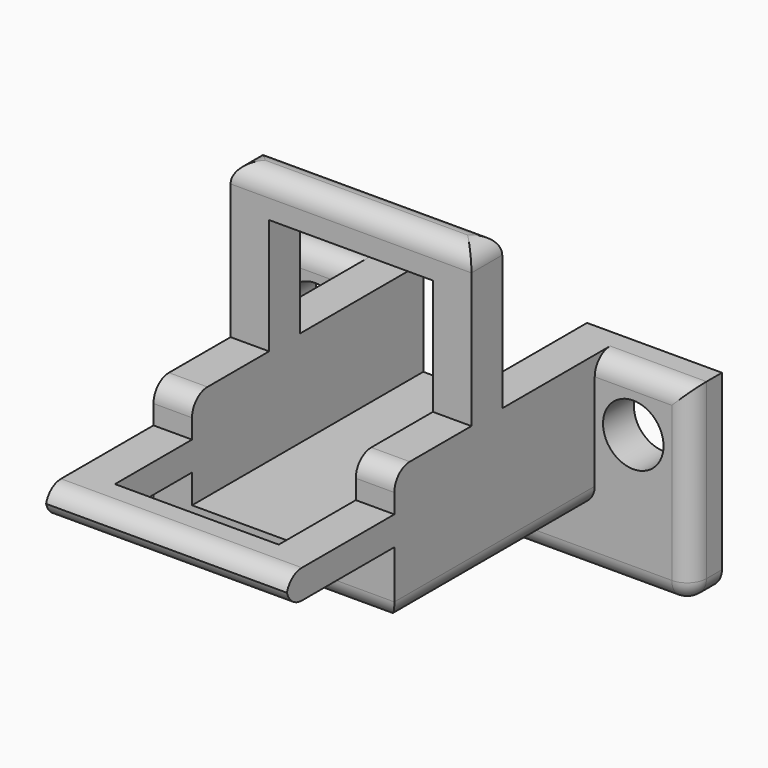
from build123d import *

# Parameters (mm, degrees)
F1_DEPTH      = 19.05
F0_R          = 1.9939
F2_DEPTH      = 2.54
F3_W          = 2.54
F3_H          = 1.905
F4_DEPTH      = 8.89
F5_W          = 2.54
F5_H          = 1.905
F6_DEPTH      = 11.43
F7_W          = 2.54
F7_H          = 2.54
F8_W          = 2.54
F8_H          = 2.54
F9_DEPTH      = 10.16
F10_W         = 2.54
F10_H         = 2.54
F11_DEPTH     = 11.43
F12_T1_DEPTH  = 9.525
F12_T3_DEPTH  = 14.605
F12_T5_DEPTH  = 26.035
F12_T7_DEPTH  = 9.525
F12_T9_DEPTH  = 4.445
F12_T11_DEPTH = 19.685
F12_T13_DEPTH = 22.225
F12_T15_DEPTH = 8.89
F12_T17_DEPTH = 8.89
F12_T19_DEPTH = 8.89
F12_S23_W     = 1.27
F12_S23_H     = 1.27
F12_T24_DEPTH = 1.27
F12_S29_W     = 1.27
F12_S29_H     = 1.27
F12_T30_DEPTH = 1.27


# Not quite as in the source:
# - a fillet or chamfer that OpenCascade refuses, or shapes differently, is made with other operations: its cross-section is extruded or revolved along the edge and cut away or added


with BuildPart() as f1:
    # F0 (on Front) → F1 (new body)
    with BuildSketch(Plane.XZ):
        Polygon((-23.2056408978, -6.35), (-23.2056408978, 0), (-25.7456408978, 0), (-25.7456408978, -8.89), (-9.8706408978, -8.89), (-9.8706408978, 0), (-12.4106408978, 0), (-12.4106408978, -6.35), align=None)
    extrude(amount=F1_DEPTH)

    # F0 (on Front) → F2 (join)
    with BuildSketch(Plane.XZ):
        Polygon((-25.7456408978, -8.89), (-25.7456408978, 0), (-32.0956408978, 0), (-32.0956408978, -12.7), (-3.5206408978, -12.7), (-3.5206408978, 0), (-9.8706408978, 0), (-9.8706408978, -8.89), align=None)
        Polygon((-28.6261399051, -11.2280230969), (-28.955778145, -11.2280230969), (-29.2968038878, -10.3571788012), (-30.3941995557, -10.3571788012), (-30.7310299027, -11.2280230969), (-31.0534760356, -11.2280230969), (-29.9710639241, -8.4782408335), (-29.7031579363, -8.4782408335), align=None, mode=Mode.SUBTRACT)
        with Locations((-28.2856408978, -3.81)):
            Circle(F0_R, mode=Mode.SUBTRACT)
        with Locations((-7.3306408978, -3.81)):
            Circle(F0_R, mode=Mode.SUBTRACT)
    extrude(amount=F2_DEPTH)

    # F3 (on face) → F4 (join)
    with BuildSketch(Plane.XZ.offset(19.05)):
        with Locations((-11.1406408978, -3.4925)):
            Rectangle(F3_W, F3_H)
        with Locations((-24.4756408978, -3.4925)):
            Rectangle(F3_W, F3_H)
    extrude(amount=F4_DEPTH)

    # F5 (on face) → F6 (join)
    with BuildSketch(Plane(origin=(-12.4106408978, 0, 0), x_dir=(0, -1, 0), z_dir=(-1, 0, 0))):
        with Locations((26.67, -3.4925)):
            Rectangle(F5_W, F5_H)
    extrude(amount=F6_DEPTH)

    # F7 (on face) + F8 (on face) → F9 (join)
    with BuildSketch(Plane.XY):
        with Locations((-24.4756408978, -11.43)):
            Rectangle(F7_W, F7_H)
    with BuildSketch(Plane.XY):
        with Locations((-11.1406408978, -11.43)):
            Rectangle(F8_W, F8_H)
    extrude(amount=F9_DEPTH)

    # F10 (on face) → F11 (join)
    with BuildSketch(Plane.YZ.offset(-23.2056408978)):
        with Locations((-11.43, 8.89)):
            Rectangle(F10_W, F10_H)
    extrude(amount=F11_DEPTH)

    # F12: fillet of radius 1.27 on 18 edges, made by hand

    # F12_s2 → F12_t1 (cut)
    with BuildSketch(Plane.YZ.offset(-35.2706408978)):
        with BuildLine():
            ThreePointArc((-1.27, 0), (-2.1680256121, -0.3719743879), (-2.54, -1.27))
            Line((-2.54, -1.27), (-2.54, 0))
            Line((-2.54, 0), (-1.27, 0))
        make_face()
    extrude(amount=F12_T1_DEPTH, mode=Mode.SUBTRACT)

    # F12_s4 → F12_t3 (cut)
    with BuildSketch(Plane.XY.offset(-11.43)):
        with BuildLine():
            ThreePointArc((-32.0956408978, -1.27), (-31.7236665099, -2.1680256121), (-30.8256408978, -2.54))
            Line((-30.8256408978, -2.54), (-32.0956408978, -2.54))
            Line((-32.0956408978, -2.54), (-32.0956408978, -1.27))
        make_face()
        with BuildLine():
            ThreePointArc((-3.5206408978, -1.27), (-3.8926152856, -2.1680256121), (-4.7906408978, -2.54))
            Line((-4.7906408978, -2.54), (-3.5206408978, -2.54))
            Line((-3.5206408978, -2.54), (-3.5206408978, -1.27))
        make_face()
    extrude(amount=F12_T3_DEPTH, mode=Mode.SUBTRACT)

    # F12_s6 → F12_t5 (cut)
    with BuildSketch(Plane.YZ.offset(-30.8256408978)):
        with BuildLine():
            ThreePointArc((-1.27, -12.7), (-2.1680256121, -12.3280256121), (-2.54, -11.43))
            Line((-2.54, -11.43), (-2.54, -12.7))
            Line((-2.54, -12.7), (-1.27, -12.7))
        make_face()
    extrude(amount=F12_T5_DEPTH, mode=Mode.SUBTRACT)

    # F12_s8 → F12_t7 (cut)
    with BuildSketch(Plane.YZ.offset(-9.8706408978)):
        with BuildLine():
            ThreePointArc((-1.27, 0), (-2.1680256121, -0.3719743879), (-2.54, -1.27))
            Line((-2.54, -1.27), (-2.54, 0))
            Line((-2.54, 0), (-1.27, 0))
        make_face()
    extrude(amount=F12_T7_DEPTH, mode=Mode.SUBTRACT)

    # F12_s10 → F12_t9 (cut)
    with BuildSketch(Plane.XZ.offset(-3.175)):
        with BuildLine():
            ThreePointArc((-4.7906408978, -12.7), (-3.8926152856, -12.3280256121), (-3.5206408978, -11.43))
            Line((-3.5206408978, -11.43), (-3.5206408978, -12.7))
            Line((-3.5206408978, -12.7), (-4.7906408978, -12.7))
        make_face()
        with BuildLine():
            ThreePointArc((-32.0956408978, -11.43), (-31.7236665099, -12.3280256121), (-30.8256408978, -12.7))
            Line((-30.8256408978, -12.7), (-32.0956408978, -12.7))
            Line((-32.0956408978, -12.7), (-32.0956408978, -11.43))
        make_face()
    extrude(amount=F12_T9_DEPTH, mode=Mode.SUBTRACT)

    # F12_s12 → F12_t11 (cut)
    with BuildSketch(Plane.XZ.offset(2.54)):
        with BuildLine():
            ThreePointArc((-9.8706408978, -7.62), (-10.2426152856, -8.5180256121), (-11.1406408978, -8.89))
            Line((-11.1406408978, -8.89), (-9.8706408978, -8.89))
            Line((-9.8706408978, -8.89), (-9.8706408978, -7.62))
        make_face()
        with BuildLine():
            ThreePointArc((-25.7456408978, -7.62), (-25.3736665099, -8.5180256121), (-24.4756408978, -8.89))
            Line((-24.4756408978, -8.89), (-25.7456408978, -8.89))
            Line((-25.7456408978, -8.89), (-25.7456408978, -7.62))
        make_face()
    extrude(amount=F12_T11_DEPTH, mode=Mode.SUBTRACT)

    # F12_s14 → F12_t13 (cut)
    with BuildSketch(Plane.YZ.offset(-28.9206408978)):
        with BuildLine():
            ThreePointArc((-26.67, -2.54), (-27.5680256121, -2.9119743879), (-27.94, -3.81))
            Line((-27.94, -3.81), (-27.94, -2.54))
            Line((-27.94, -2.54), (-26.67, -2.54))
        make_face()
        with BuildLine():
            ThreePointArc((-19.05, -7.62), (-18.6780256121, -8.5180256121), (-17.78, -8.89))
            Line((-17.78, -8.89), (-19.05, -8.89))
            Line((-19.05, -8.89), (-19.05, -7.62))
        make_face()
        with BuildLine():
            ThreePointArc((-27.94, -3.175), (-27.5680256121, -4.0730256121), (-26.67, -4.445))
            Line((-26.67, -4.445), (-27.94, -4.445))
            Line((-27.94, -4.445), (-27.94, -3.175))
        make_face()
        with BuildLine():
            ThreePointArc((-11.43, 10.16), (-12.3280256121, 9.7880256121), (-12.7, 8.89))
            Line((-12.7, 8.89), (-12.7, 10.16))
            Line((-12.7, 10.16), (-11.43, 10.16))
        make_face()
        with BuildLine():
            ThreePointArc((-10.16, 8.89), (-10.5319743879, 9.7880256121), (-11.43, 10.16))
            Line((-11.43, 10.16), (-10.16, 10.16))
            Line((-10.16, 10.16), (-10.16, 8.89))
        make_face()
    extrude(amount=F12_T13_DEPTH, mode=Mode.SUBTRACT)

    # F12_s16 → F12_t15 (cut)
    with BuildSketch(Plane.YZ.offset(-28.9206408978)):
        with BuildLine():
            ThreePointArc((-19.05, -1.27), (-18.6780256121, -0.3719743879), (-17.78, 0))
            Line((-17.78, 0), (-19.05, 0))
            Line((-19.05, 0), (-19.05, -1.27))
        make_face()
    extrude(amount=F12_T15_DEPTH, mode=Mode.SUBTRACT)

    # F12_s18 → F12_t17 (cut)
    with BuildSketch(Plane.YZ.offset(-15.5856408978)):
        with BuildLine():
            ThreePointArc((-17.78, 0), (-18.6780256121, -0.3719743879), (-19.05, -1.27))
            Line((-19.05, -1.27), (-19.05, 0))
            Line((-19.05, 0), (-17.78, 0))
        make_face()
    extrude(amount=F12_T17_DEPTH, mode=Mode.SUBTRACT)

    # F12_s20 → F12_t19 (cut)
    with BuildSketch(Plane.XZ.offset(6.985)):
        with BuildLine():
            ThreePointArc((-25.7456408978, 8.89), (-25.3736665099, 9.7880256121), (-24.4756408978, 10.16))
            Line((-24.4756408978, 10.16), (-25.7456408978, 10.16))
            Line((-25.7456408978, 10.16), (-25.7456408978, 8.89))
        make_face()
        with BuildLine():
            ThreePointArc((-9.8706408978, 8.89), (-10.2426152856, 9.7880256121), (-11.1406408978, 10.16))
            Line((-11.1406408978, 10.16), (-9.8706408978, 10.16))
            Line((-9.8706408978, 10.16), (-9.8706408978, 8.89))
        make_face()
    extrude(amount=F12_T19_DEPTH, mode=Mode.SUBTRACT)


with BuildPart() as f12_tool22:
    # F12_s23 → F12_t24 (new body)
    with BuildSketch(Plane.YZ.offset(-30.8256408978)):
        with Locations((-1.905, -12.065)):
            Rectangle(F12_S23_W, F12_S23_H)
    extrude(amount=-F12_T24_DEPTH)

    # F12_s25 → F12_t26 (revolve, cut)
    with BuildSketch(Plane(origin=(-30.8256408978, -1.27, -11.43), x_dir=(0, 0.7071067812, 0.7071067812), z_dir=(0, -0.7071067812, 0.7071067812))):
        with BuildLine():
            ThreePointArc((0, -1.27), (1.27, 0), (0, 1.27))
            Line((0, 1.27), (0, -1.27))
        make_face()
    revolve(axis=Axis((-30.8256408978, -1.27, -11.43), (-1, 0, 0)), mode=Mode.SUBTRACT)


with BuildPart() as f1_1:
    add(f1.part)

    # F12_t21: cut F12_tool22
    add(f12_tool22.part, mode=Mode.SUBTRACT)


with BuildPart() as f12_tool28:
    # F12_s29 → F12_t30 (new body)
    with BuildSketch(Plane.YZ.offset(-4.7906408978)):
        with Locations((-1.905, -12.065)):
            Rectangle(F12_S29_W, F12_S29_H)
    extrude(amount=F12_T30_DEPTH)

    # F12_s31 → F12_t32 (revolve, cut)
    with BuildSketch(Plane(origin=(-4.7906408978, -1.27, -11.43), x_dir=(0, 0.7071067812, 0.7071067812), z_dir=(0, 0.7071067812, -0.7071067812))):
        with BuildLine():
            ThreePointArc((0, -1.27), (1.27, 0), (0, 1.27))
            Line((0, 1.27), (0, -1.27))
        make_face()
    revolve(axis=Axis((-4.7906408978, -1.27, -11.43), (1, 0, 0)), mode=Mode.SUBTRACT)


with BuildPart() as f1_2:
    add(f1_1.part)

    # F12_t27: cut F12_tool28
    add(f12_tool28.part, mode=Mode.SUBTRACT)


solid = f1_2.part
